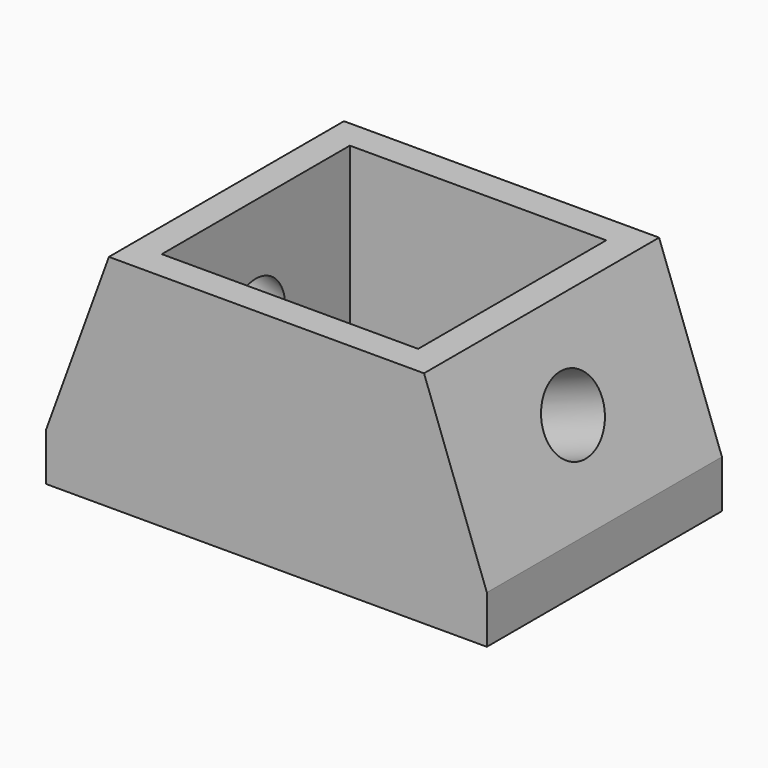
from build123d import *

# Parameters (mm, degrees)
F0_W     = 76.2
F0_H     = 50.8
F1_DEPTH = 38.1
F3_DEPTH = 50.8
F4_W     = 44.3217208988
F4_H     = 40.64
F5_DEPTH = 27.8086844974
F6_R     = 6.35
F7_DEPTH = 13.4962615407
F8_R     = 6.35
F9_DEPTH = 13.4962615407


with BuildPart() as f1:
    # F0 (on Top) → F1 (new body)
    with BuildSketch(Plane.XY):
        with Locations((38.1, 25.4)):
            Rectangle(F0_W, F0_H)
    extrude(amount=F1_DEPTH)

    # F2 (on face) → F3 (cut, through all)
    with BuildSketch(Plane.XZ):
        Polygon((0, 38.1), (0, 8.26475929), (10.8591395506, 38.1), align=None)
        Polygon((76.2, 38.1), (65.3408604494, 38.1), (76.2, 8.26475929), align=None)
    extrude(amount=-F3_DEPTH, mode=Mode.SUBTRACT)

    # F4 (on face) → F5 (cut, through all)
    with BuildSketch(Plane.XY.offset(38.1)):
        with Locations((38.1, 25.4)):
            Rectangle(F4_W, F4_H)
    extrude(amount=-F5_DEPTH, mode=Mode.SUBTRACT)

    # F6 (on face) → F7 (cut, through all)
    with BuildSketch(Plane(origin=(-2.6562424343, 0, 0.9667931811), x_dir=(0, -1, 0), z_dir=(-0.9396926208, 0, 0.3420201433))):
        with Locations((-25.4, 23.6413333174)):
            Circle(F6_R)
    extrude(amount=-F7_DEPTH, mode=Mode.SUBTRACT)

    # F8 (on face) → F9 (cut, through all)
    with BuildSketch(Plane(origin=(69.9425357172, 0, 25.4570011102), x_dir=(0, 1, 0), z_dir=(0.9396926208, 0, 0.3420201433))):
        with Locations((25.4, -2.420601604)):
            Circle(F8_R)
    extrude(amount=-F9_DEPTH, mode=Mode.SUBTRACT)


solid = f1.part
